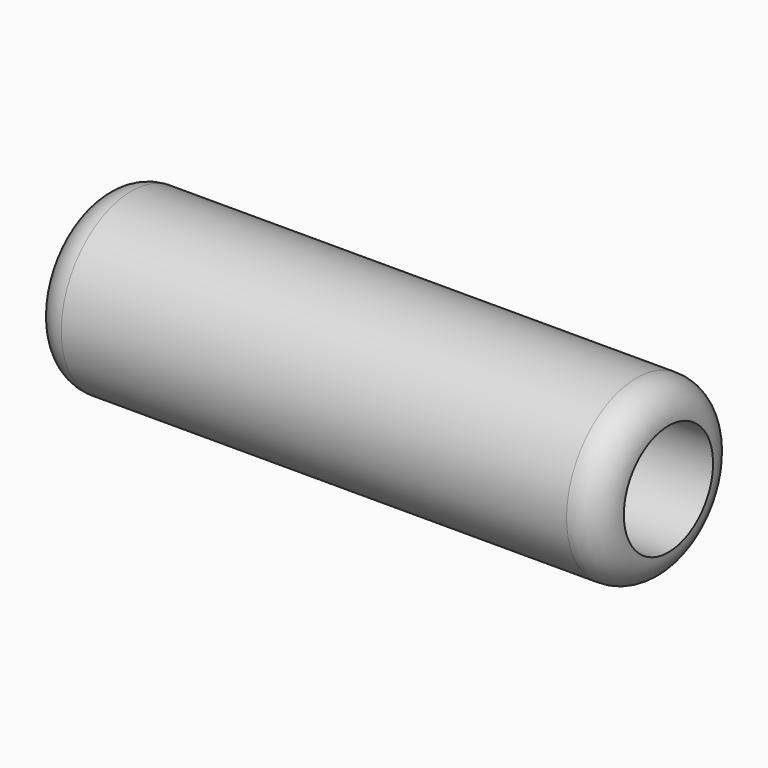
from build123d import *

# Parameters (mm, degrees)
F2_R = 6.34999


# Not quite as in the source:
# - a fillet or chamfer is up to 0.001 mm smaller than in the source, because OpenCascade refuses the exact size


with BuildPart() as f1:
    # F0 (on Front) → F1 (revolve)
    with BuildSketch(Plane.XZ):
        Polygon((3.9624, -2.38125), (0, -2.38125), (0, -19.85645), (113.5126, -19.85645), (113.5126, -13.50645), (3.9624, -13.50645), align=None)
    revolve(axis=Axis((1.9812, 0, -2.38125), (-1, 0, 0)))

    # F2 (radius 6.35 in the source; OpenCascade refuses exactly that, so slightly less here)
    f2_edges = [f1.edges().sort_by_distance(p)[0] for p in [
        (0, 0, 15.09395),
        (113.5126, 0, 15.09395),
        (56.7563, 0, -19.85645),
    ]]
    fillet(f2_edges, radius=F2_R)


solid = f1.part
